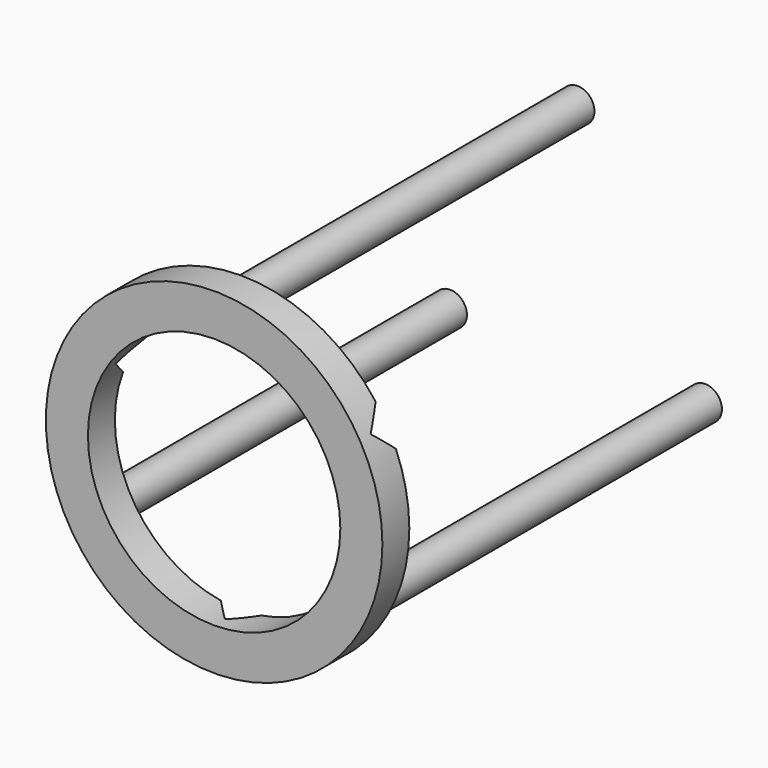
from build123d import *

# Parameters (mm, degrees)
F0_R            = 10
F0_R_2          = 7.5
F1_DEPTH        = 2
F3_DEPTH        = 25
F3_COPIES_COUNT = 3
F4_R            = 1
F5_DEPTH        = 25
F5_COPIES_COUNT = 3


# Not quite as in the source:
# - a pattern or mirror of a feature is missing from the dataset's text; its kind, count and spacing are read off the source's solid


with BuildPart() as f1:
    # F0 (on Front) → F1 (new body)
    with BuildSketch(Plane.XZ):
        Circle(F0_R)
        Circle(F0_R_2, mode=Mode.SUBTRACT)
    extrude(amount=F1_DEPTH)

    # F2 (on Top) → F3 (cut)
    with BuildSketch(Plane.XY):
        Polygon((-1.2, 0), (0, -1.2), (1.2, 0), align=None)
    f3 = extrude(amount=-F3_DEPTH, mode=Mode.SUBTRACT)

    # F3_copies: F3 ×3 about axis
    f3_copies_axis = Axis((0, 0, 0), (0, 1, 0))
    for i in range(1, F3_COPIES_COUNT):
        add(f3.rotate(f3_copies_axis, i * 360 / F3_COPIES_COUNT), mode=Mode.SUBTRACT)

    # F4 (on Front) → F5 (join)
    with BuildSketch(Plane.XZ):
        with Locations((0, 8.75)):
            Circle(F4_R)
    f5 = extrude(amount=-F5_DEPTH)

    # F5_copies: F5 ×3 about axis
    f5_copies_axis = Axis((0, 0, 0), (0, 1, 0))
    for i in range(1, F5_COPIES_COUNT):
        add(f5.rotate(f5_copies_axis, i * 360 / F5_COPIES_COUNT))


solid = f1.part
